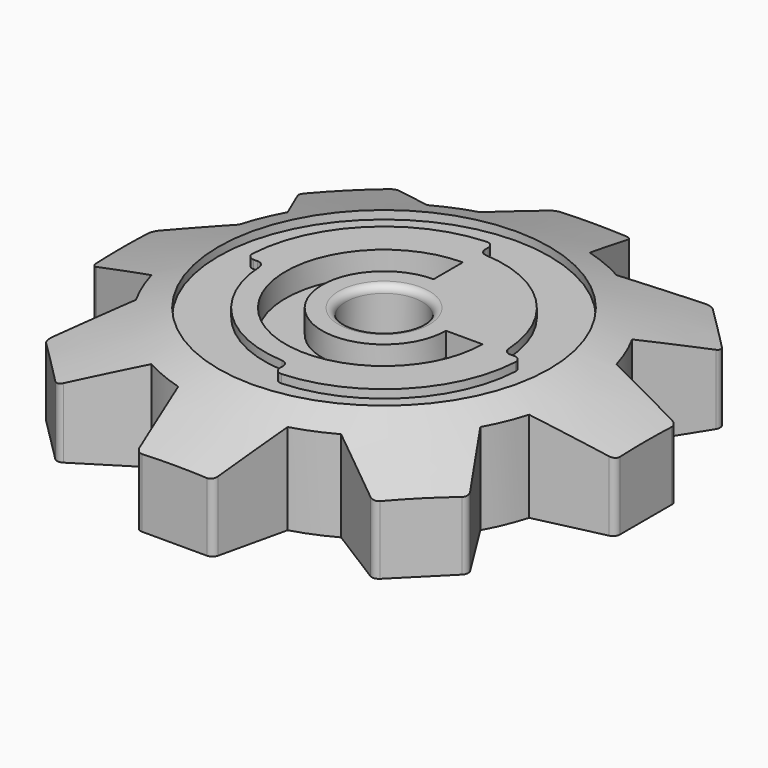
from build123d import *

# Parameters (mm, degrees)
F1_DEPTH = 14.478
F5_R     = 23.6640826147
F6_DEPTH = 1.1938
F5_R_2   = 5.4611807343
F7_DEPTH = 18.034
F8_DEPTH = 3.3782
F9_R     = 1.016


with BuildPart() as f1:
    # F0 (on Top) → F1 (new body)
    with BuildSketch(Plane.XY):
        with BuildLine():
            Line((-30.3200407773, 22.6429850771), (-24.6294784274, 13.5667208411))
            ThreePointArc((-24.6294784274, 13.5667208411), (-25.9783872248, 10.7606003171), (-27.0087915183, 7.8225509079))
            Line((-27.0087915183, 7.8225509079), (-37.4505147338, 5.4284981452))
            Line((-37.4505147338, 5.4284981452), (-37.4505147338, -5.4284981452))
            Line((-37.4505147338, -5.4284981452), (-27.0087915183, -7.8225509079))
            ThreePointArc((-27.0087915183, -7.8225509079), (-25.9783872248, -10.7606003171), (-24.6294784274, -13.5667208411))
            Line((-24.6294784274, -13.5667208411), (-30.3200407773, -22.6429850771))
            Line((-30.3200407773, -22.6429850771), (-22.6429850771, -30.3200407773))
            Line((-22.6429850771, -30.3200407773), (-13.5667208411, -24.6294784274))
            ThreePointArc((-13.5667208411, -24.6294784274), (-10.7606003171, -25.9783872248), (-7.8225509079, -27.0087915183))
            Line((-7.8225509079, -27.0087915183), (-5.4284981452, -37.4505147338))
            Line((-5.4284981452, -37.4505147338), (5.4284981452, -37.4505147338))
            Line((5.4284981452, -37.4505147338), (7.8225509079, -27.0087915183))
            ThreePointArc((7.8225509079, -27.0087915183), (10.7606003171, -25.9783872248), (13.5667208411, -24.6294784274))
            Line((13.5667208411, -24.6294784274), (22.6429850771, -30.3200407773))
            Line((22.6429850771, -30.3200407773), (30.3200407773, -22.6429850771))
            Line((30.3200407773, -22.6429850771), (24.6294784274, -13.5667208411))
            ThreePointArc((24.6294784274, -13.5667208411), (25.9783872248, -10.7606003171), (27.0087915183, -7.8225509079))
            Line((27.0087915183, -7.8225509079), (37.4505147338, -5.4284981452))
            Line((37.4505147338, -5.4284981452), (37.4505147338, 5.4284981452))
            Line((37.4505147338, 5.4284981452), (27.0087915183, 7.8225509079))
            ThreePointArc((27.0087915183, 7.8225509079), (25.9783872248, 10.7606003171), (24.6294784274, 13.5667208411))
            Line((24.6294784274, 13.5667208411), (30.3200407773, 22.6429850771))
            Line((30.3200407773, 22.6429850771), (22.6429850771, 30.3200407773))
            Line((22.6429850771, 30.3200407773), (13.5667208411, 24.6294784274))
            ThreePointArc((13.5667208411, 24.6294784274), (10.7606003171, 25.9783872248), (7.8225509079, 27.0087915183))
            Line((7.8225509079, 27.0087915183), (5.4284981452, 37.4505147338))
            Line((5.4284981452, 37.4505147338), (-5.4284981452, 37.4505147338))
            Line((-5.4284981452, 37.4505147338), (-7.8225509079, 27.0087915183))
            ThreePointArc((-7.8225509079, 27.0087915183), (-10.7606003171, 25.9783872248), (-13.5667208411, 24.6294784274))
            Line((-13.5667208411, 24.6294784274), (-22.6429850771, 30.3200407773))
            Line((-22.6429850771, 30.3200407773), (-30.3200407773, 22.6429850771))
        make_face()
    extrude(amount=F1_DEPTH)

    # F3 (on Front) → F4 (revolve, cut)
    with BuildSketch(Plane.XZ):
        Polygon((-39.187733084, 17.5162125379), (-39.187733084, 9.2955380678), (-23.6767126761, 14.478), (-23.6767126761, 17.5162125379), align=None)
    revolve(axis=Axis((0, 0, 21.3634204119), (0, 0, 1)), mode=Mode.SUBTRACT)

    # F5 (on face) → F6 (cut)
    with BuildSketch(Plane.XY.offset(14.478)):
        Circle(F5_R)
        with BuildLine():
            ThreePointArc((-19.6771575376, 0), (-13.9138515293, 13.9138515293), (0, 19.6771575376))
            Line((0, 19.6771575376), (0, 17.0739562129))
            ThreePointArc((0, 17.0739562129), (12.0731102199, 12.0731102199), (17.0739562129, 0))
            Line((17.0739562129, 0), (19.6771575376, 0))
            ThreePointArc((19.6771575376, 0), (13.9138515293, -13.9138515293), (0, -19.6771575376))
            Line((0, -19.6771575376), (0, -17.0739562129))
            ThreePointArc((0, -17.0739562129), (-12.0731102199, -12.0731102199), (-17.0739562129, 0))
            Line((-17.0739562129, 0), (-19.6771575376, 0))
        make_face(mode=Mode.SUBTRACT)
    extrude(amount=-F6_DEPTH, mode=Mode.SUBTRACT)

    # F5 (on face) → F7 (cut)
    with BuildSketch(Plane.XY.offset(14.478)):
        Circle(F5_R_2)
    extrude(amount=-F7_DEPTH, mode=Mode.SUBTRACT)

    # F5 (on face) → F8 (cut)
    with BuildSketch(Plane.XY.offset(14.478)):
        with BuildLine():
            Line((0, 8.8564318695), (0, 14.0838984666))
            ThreePointArc((0, 14.0838984666), (-9.9588201113, -9.9588201113), (14.0838984666, 0))
            Line((14.0838984666, 0), (8.8564318695, 0))
            ThreePointArc((8.8564318695, 0), (-6.262443032, -6.262443032), (0, 8.8564318695))
        make_face()
    extrude(amount=-F8_DEPTH, mode=Mode.SUBTRACT)

    # F9
    f9_edges = [f1.edges().sort_by_distance(p)[0] for p in [
        (-37.450515, -5.428498, 4.8726),
        (-37.450515, 5.428498, 4.8726),
        (-30.320041, -22.642985, 4.8726),
        (-22.642985, -30.320041, 4.8726),
        (-5.428498, -37.450515, 4.8726),
        (5.428498, -37.450515, 4.8726),
        (22.642985, -30.320041, 4.8726),
        (30.320041, -22.642985, 4.8726),
        (37.450515, -5.428498, 4.8726),
        (37.450515, 5.428498, 4.8726),
        (30.320041, 22.642985, 4.8726),
        (22.642985, 30.320041, 4.8726),
        (5.428498, 37.450515, 4.8726),
        (-5.428498, 37.450515, 4.8726),
        (-30.320041, 22.642985, 4.8726),
        (-22.642985, 30.320041, 4.8726),
        (19.677158, 0, 13.8811),
        (17.073956, 0, 13.8811),
        (0, 17.073956, 13.8811),
        (0, 19.677158, 13.8811),
        (-5.461181, 0, 14.478),
        (-19.677158, 0, 13.8811),
        (-17.073956, 0, 13.8811),
        (0, -19.677158, 13.8811),
        (0, -17.073956, 13.8811),
    ]]
    fillet(f9_edges, radius=F9_R)


solid = f1.part
